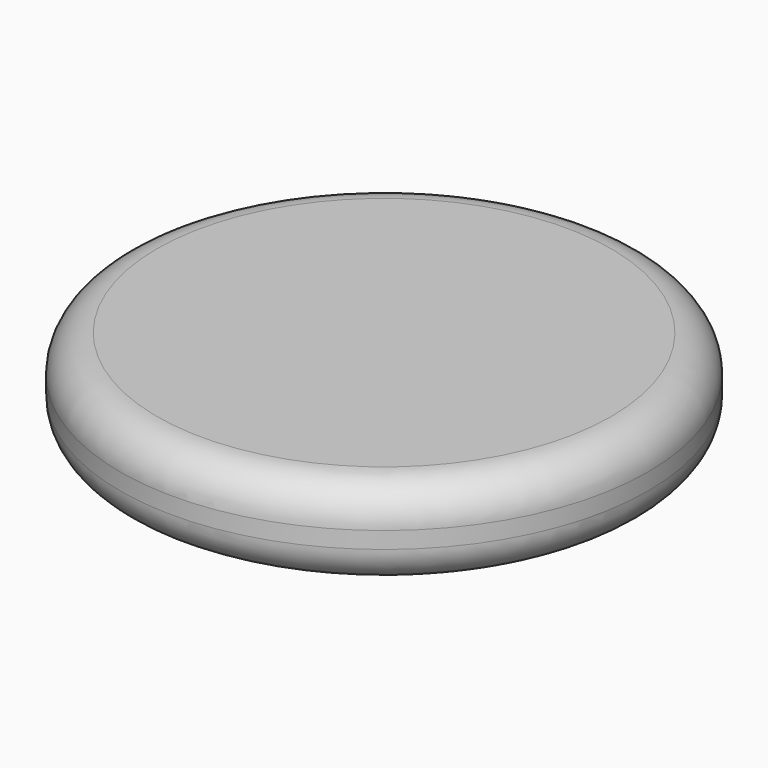
from build123d import *

# Parameters (mm, degrees)
F0_R     = 22.5
F0_R_2   = 13.3867529453
F1_DEPTH = 7.7
F2_R     = 3.1384776311
F3_DEPTH = 3


# Not quite as in the source:
# - a fillet or chamfer that OpenCascade refuses, or shapes differently, is made with other operations: its cross-section is extruded or revolved along the edge and cut away or added


with BuildPart() as f1:
    # F0 (on Top) → F1 (new body)
    with BuildSketch(Plane.XY):
        with Locations((-30.7742264122, 10.8950231224)):
            Circle(F0_R)
        with Locations((-30.7742264122, 10.8950231224)):
            Circle(F0_R_2, mode=Mode.SUBTRACT)
    extrude(amount=-F1_DEPTH)

    # F2
    f2_edges = [f1.edges().sort_by_distance(p)[0] for p in [
        (-8.274226, 10.895023, -3.85),
        (-53.274226, 10.895023, 0),
        (-53.274226, 10.895023, -7.7),
    ]]
    fillet(f2_edges, radius=F2_R)

    # F0 (on Top) → F3 (join)
    with BuildSketch(Plane.XY):
        with Locations((-30.7742264122, 10.8950231224)):
            Circle(F0_R_2)
    extrude(amount=-F3_DEPTH)

    # F4: fillet of radius 5 on 1 edges, made by hand

    # F4_s1 → F4_t2 (revolve)
    with BuildSketch(Plane.XZ.offset(-10.8950231224)):
        with BuildLine():
            ThreePointArc((-17.3874734669, -7.7), (-18.9506380521, -4.3599450554), (-22.3784653523, -3))
            Line((-22.3784653523, -3), (-17.3874734669, -3))
            Line((-17.3874734669, -3), (-17.3874734669, -7.7))
        make_face()
    revolve(axis=Axis((-30.7742264122, 10.8950231224, -3), (0, 0, 1)))


solid = f1.part
